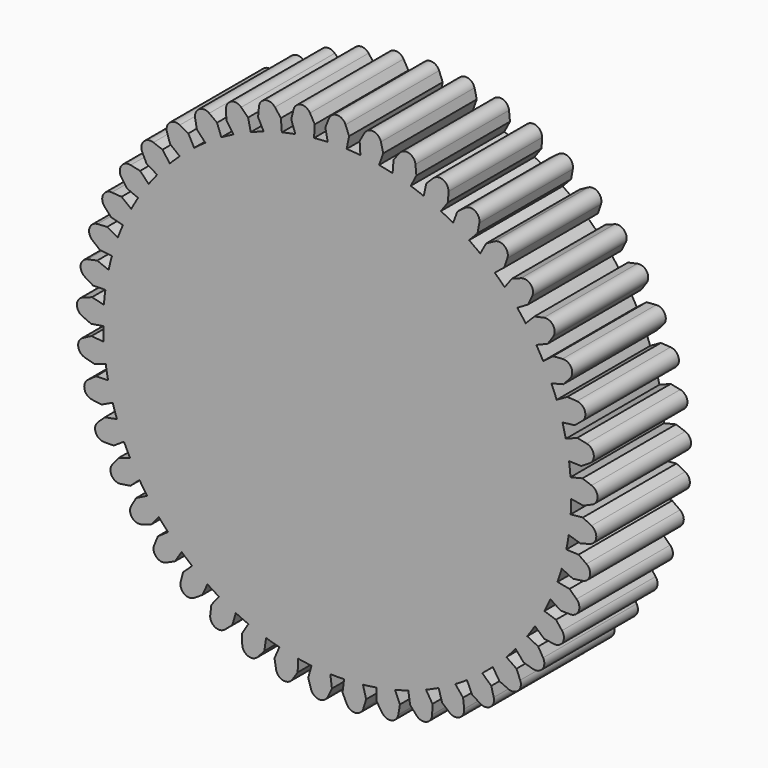
from build123d import *

# Parameters (mm, degrees)
F0_R            = 50.8
F1_DEPTH        = 25.4
F3_DEPTH        = 25.4
F3_COPIES_COUNT = 45


# Not quite as in the source:
# - a pattern or mirror of a feature is missing from the dataset's text; its kind, count and spacing are read off the source's solid


with BuildPart() as f1:
    # F0 (on Front) → F1 (new body)
    with BuildSketch(Plane.XZ):
        Circle(F0_R)
    extrude(amount=F1_DEPTH)

    # F2 (on Front) → F3 (join)
    with BuildSketch(Plane.XZ):
        with BuildLine():
            ThreePointArc((-2.0394499691, 50.7132378554), (0, 50.7962406895), (2.0394499691, 50.7132378554))
            Line((2.0394499691, 50.7132378554), (2.5789397816, 53.3691877014))
            Line((2.5789397816, 53.3691877014), (1.8071979284, 55.324267596))
            ThreePointArc((1.8071979284, 55.324267596), (0, 56.5537994158), (-1.8071979284, 55.324267596))
            Line((-1.8071979284, 55.324267596), (-2.5789397816, 53.3691877014))
            Line((-2.5789397816, 53.3691877014), (-2.0394499691, 50.7132378554))
        make_face()
    f3 = extrude(amount=F3_DEPTH)

    # F3_copies: F3 ×45 about axis
    f3_copies_axis = Axis((0, 0, 0), (0, 1, 0))
    for i in range(1, F3_COPIES_COUNT):
        add(f3.rotate(f3_copies_axis, i * 360 / F3_COPIES_COUNT))


with BuildPart() as f5_1:
    # F5: copy of F1
    add(f1.part)


solid = f1.part
